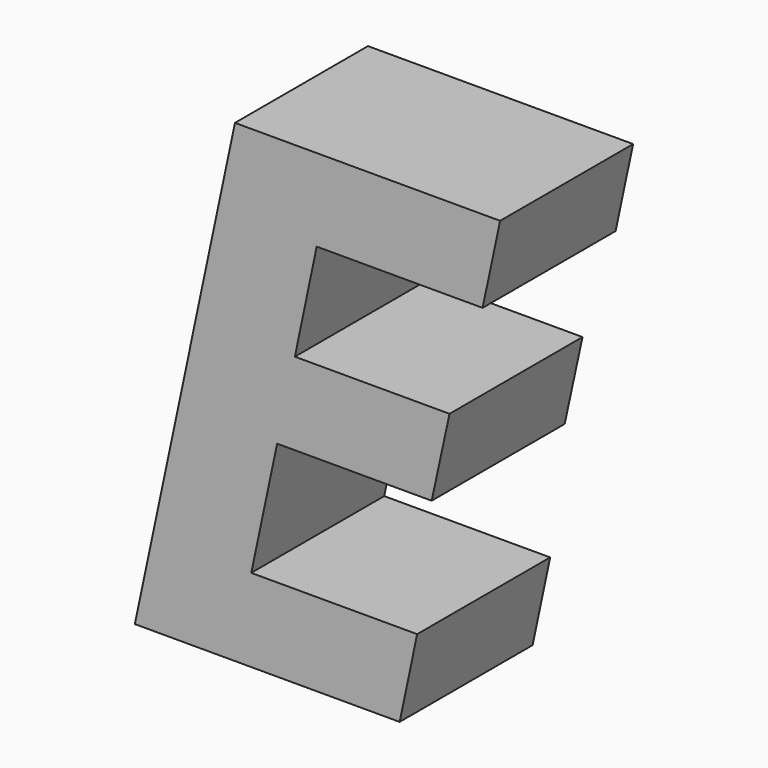
from build123d import *

# Parameters (mm, degrees)
F0_TEXT_SIZE = 101.4068800335
F1_DEPTH     = 25.4


# Not quite as in the source:
# - Text() gives the source's letters only with a copy of the font that has no kerning and outlines rounded to 1/6400 em; it was checked with that copy


with BuildPart() as f1:
    # F0 (on Front) → F1 (new body)
    with BuildSketch(Plane.XZ):
        with Locations((-48.6286729574, -50.1014366746)):
            Text('E', F0_TEXT_SIZE, font='Open Sans', font_style=FontStyle.BOLDITALIC, text_align=(TextAlign.LEFT, TextAlign.BOTTOM))
    extrude(amount=F1_DEPTH)


solid = f1.part
